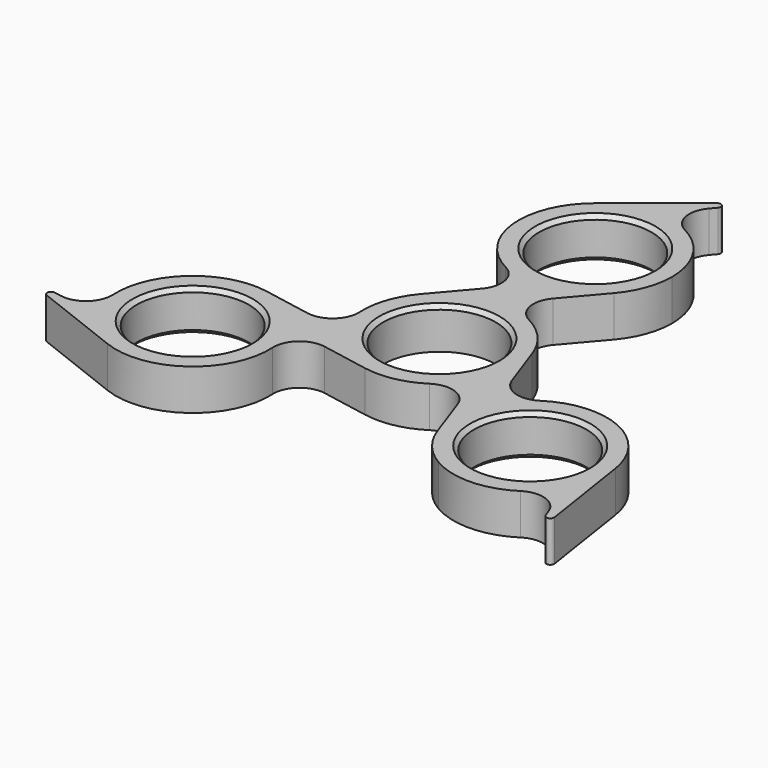
from build123d import *

# Parameters (mm, degrees)
F0_R            = 11
F1_DEPTH        = 8
F2_DEPTH        = 8
F2_COPIES_COUNT = 3
F3_R            = 5.08
F4_F1_R         = 0.762
F4_F2_R         = 0.762
F4_F3_R         = 0.762
F5_SIZE         = 0.762


# Not quite as in the source:
# - a pattern or mirror of a feature is missing from the dataset's text; its kind, count and spacing are read off the source's solid


with BuildPart() as f1:
    # F0 (on Top) → F1 (new body)
    with BuildSketch(Plane.XY):
        with BuildLine():
            ThreePointArc((-11.407337121, 9.7402597403), (-5.190854611, -14.0732024929), (15, 0))
            ThreePointArc((15, 0), (10.6066017178, 10.6066017178), (0, 15))
            ThreePointArc((0, 15), (-6.2807684202, 13.6217454114), (-11.407337121, 9.7402597403))
        make_face()
        Circle(F0_R, mode=Mode.SUBTRACT)
    extrude(amount=-F1_DEPTH)

    # F0 (on Top) → F2 (join, through all)
    with BuildSketch(Plane.XY):
        with BuildLine():
            ThreePointArc((-11.407337121, 9.7402597403), (-6.2807684202, 13.6217454114), (0, 15))
            Line((0, 15), (11.407337121, 28.3597402597))
            ThreePointArc((11.407337121, 28.3597402597), (6.2807684202, 24.4782545886), (0, 23.1))
            Line((0, 23.1), (-11.407337121, 9.7402597403))
        make_face()
        with BuildLine():
            ThreePointArc((0, 23.1), (6.2807684202, 24.4782545886), (11.407337121, 28.3597402597))
            ThreePointArc((11.407337121, 28.3597402597), (14.0732024929, 32.909145389), (15, 38.1))
            ThreePointArc((15, 38.1), (10.6066017178, 48.7066017178), (0, 53.1))
            ThreePointArc((0, 53.1), (-4.9701878524, 52.2526404855), (-9.378837576, 49.806297695))
            ThreePointArc((-9.378837576, 49.806297695), (-14.1526404855, 33.1298121476), (0, 23.1))
        make_face()
        with Locations((0, 38.1)):
            Circle(F0_R, mode=Mode.SUBTRACT)
        with BuildLine():
            Line((11.407337121, 66.4597402597), (-9.378837576, 49.806297695))
            ThreePointArc((-9.378837576, 49.806297695), (-4.9701878524, 52.2526404855), (0, 53.1))
            Line((0, 53.1), (11.407337121, 66.4597402597))
        make_face()
    f2 = extrude(amount=-F2_DEPTH)

    # F2_copies: F2 ×3 about axis
    f2_copies_axis = Axis((0, 0, 0), (0, 0, 1))
    for i in range(1, F2_COPIES_COUNT):
        add(f2.rotate(f2_copies_axis, i * 360 / F2_COPIES_COUNT))

    # F3
    f3_edges = [f1.edges().sort_by_distance(p)[0] for p in [
        (0, 15, -4),
        (0, 23.1, -4),
        (0, 53.1, -4),
        (20.005187, -11.55, -4),
        (-12.990381, -7.5, -4),
        (-45.985949, -26.55, -4),
        (-20.005187, -11.55, -4),
        (12.990381, -7.5, -4),
        (45.985949, -26.55, -4),
    ]]
    fillet(f3_edges, radius=F3_R)

    # F4: fillet of radius 0.762 on 3 edges, made by hand

    # F4_f1
    f4_f1_edges = [f1.edges().sort_by_distance(p)[0] for p in [
        (51.8521548333, -43.1089138662, -4),
    ]]
    fillet(f4_f1_edges, radius=F4_F1_R)

    # F4_f2
    f4_f2_edges = [f1.edges().sort_by_distance(p)[0] for p in [
        (11.407337121, 66.4597402597, -4),
    ]]
    fillet(f4_f2_edges, radius=F4_F2_R)

    # F4_f3
    f4_f3_edges = [f1.edges().sort_by_distance(p)[0] for p in [
        (-63.2594919544, -23.3508263935, -4),
    ]]
    fillet(f4_f3_edges, radius=F4_F3_R)

    # F5
    f5_edges = [f1.edges().sort_by_distance(p)[0] for p in [
        (-11, 0, 0),
        (-11, 38.1, 0),
        (-11, 38.1, -8),
        (-27.495568, -28.576279, -8),
        (38.495568, -9.523721, -8),
        (-27.495568, -28.576279, 0),
        (38.495568, -9.523721, 0),
    ]]
    chamfer(f5_edges, length=F5_SIZE)


solid = f1.part
